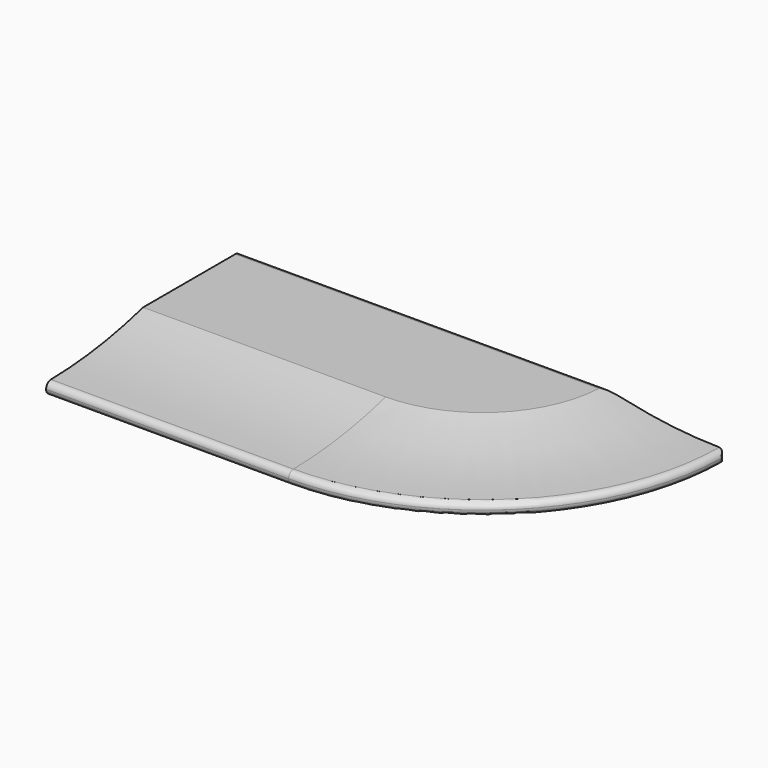
from build123d import *

# Parameters (mm, degrees)
F1_DEPTH     = 4.7625
F2_W         = 19.05
F2_H         = 6.35
F3_DEPTH     = 25.4
F4_R         = 2.54
F9_T1_DEPTH  = 9.0533559085
F9_T3_DEPTH  = 84.7725
F9_T5_DEPTH  = 53.9538612207
F9_T8_ANGLE  = 93.5585733653
F9_T10_ANGLE = 93.5585733653


# Not quite as in the source:
# - a fillet or chamfer that OpenCascade refuses, or shapes differently, is made with other operations: its cross-section is extruded or revolved along the edge and cut away or added
# - two fillets or chamfers of one size are made in one step


with BuildPart() as f1:
    # F0 (on Top) → F1 (new body, symmetric)
    with BuildSketch(Plane.XY):
        with BuildLine():
            Line((101.6, 0), (0, 0))
            Line((0, 0), (0, -50.8))
            Line((0, -50.8), (50.8, -50.8))
            ThreePointArc((50.8, -50.8), (86.7210244843, -35.9210244843), (101.6, 0))
        make_face()
    extrude(amount=F1_DEPTH, both=True)

    # F2 (on Right) → F3 (cut)
    with BuildSketch(Plane.YZ):
        with Locations((-12.7, 0)):
            Rectangle(F2_W, F2_H)
    extrude(amount=F3_DEPTH, mode=Mode.SUBTRACT)

    # F4
    f4_edges = [f1.edges().sort_by_distance(p)[0] for p in [
        (12.7, -3.175, -3.175),
        (12.7, -3.175, 3.175),
        (12.7, -22.225, -3.175),
        (12.7, -22.225, 3.175),
    ]]
    fillet(f4_edges, radius=F4_R)


with BuildPart() as f6:
    # F6: sweep along a path in F6_path
    with BuildLine(Plane(origin=(50.8, -50.8, 4.7625), x_dir=(0, 1, 0), z_dir=(0, 0, 1))) as f6_path:
        Line((0, 50.8), (0, 0))
        ThreePointArc((0, 0), (14.8789755157, -35.9210244843), (50.8, -50.8))
    # F5 (on face) → F6 (sweep)
    with BuildSketch(Plane(origin=(0, 0, 0), x_dir=(0, -1, 0), z_dir=(-1, 0, 0))):
        with BuildLine():
            Line((50.8, 4.7625), (25.4, 4.7625))
            ThreePointArc((25.4, 4.7625), (37.9805074569, 2.1472133229), (50.8, 1.27))
            Line((50.8, 1.27), (50.8, 4.7625))
        make_face()
    sweep(path=f6_path.line)


with BuildPart() as f7_1:
    # F7: instance of F6
    add(f6.part.mirror(Plane.XY))


with BuildPart() as f1_1:
    add(f1.part)

    # F8: cut F6, F7_1
    add(f6.part, mode=Mode.SUBTRACT)
    add(f7_1.part, mode=Mode.SUBTRACT)

    # F9: fillet of radius 1.27 on 8 edges, made by hand

    # F9_s2 → F9_t1 (cut)
    with BuildSketch(Plane.XY.offset(-4.5266779542)):
        with BuildLine():
            ThreePointArc((100.3137152716, 0), (101.2231811617, -0.3835623006), (101.5832977145, -1.3025641026))
            ThreePointArc((101.5832977145, -1.3025641026), (101.595824257, -0.6513355908), (101.6, 0))
            Line((101.6, 0), (100.3137152716, 0))
        make_face()
    extrude(amount=F9_T1_DEPTH, mode=Mode.SUBTRACT)

    # F9_s4 → F9_t3 (cut)
    with BuildSketch(Plane.YZ.offset(-3.175)):
        with BuildLine():
            ThreePointArc((0, 3.4925), (-0.3719743879, 4.3905256121), (-1.27, 4.7625))
            Line((-1.27, 4.7625), (0, 4.7625))
            Line((0, 4.7625), (0, 3.4925))
        make_face()
        with BuildLine():
            ThreePointArc((0, -3.4925), (-0.3719743879, -4.3905256121), (-1.27, -4.7625))
            Line((-1.27, -4.7625), (0, -4.7625))
            Line((0, -4.7625), (0, -3.4925))
        make_face()
    extrude(amount=F9_T3_DEPTH, mode=Mode.SUBTRACT)

    # F9_s6 → F9_t5 (cut)
    with BuildSketch(Plane.YZ.offset(-3.1538612207)):
        with BuildLine():
            ThreePointArc((-49.5469102739, 1.2783429251), (-50.4339845264, 0.9004824038), (-50.8, 0.0084555117))
            Line((-50.8, 0.0084555117), (-50.8, 1.27))
            ThreePointArc((-50.8, 1.27), (-50.1734412505, 1.2720857544), (-49.5469102739, 1.2783429251))
        make_face()
        with BuildLine():
            ThreePointArc((-50.8, -0.0084555117), (-50.4339845264, -0.9004824038), (-49.5469102739, -1.2783429251))
            ThreePointArc((-49.5469102739, -1.2783429251), (-50.1734412505, -1.2720857544), (-50.8, -1.27))
            Line((-50.8, -1.27), (-50.8, -0.0084555117))
        make_face()
    extrude(amount=F9_T5_DEPTH, mode=Mode.SUBTRACT)

    # F9_s7 → F9_t8 (revolve, cut)
    with BuildSketch(Plane.YZ.offset(50.8)):
        with BuildLine():
            ThreePointArc((-50.8, 0.0084555117), (-50.4339845264, 0.9004824038), (-49.5469102739, 1.2783429251))
            ThreePointArc((-49.5469102739, 1.2783429251), (-50.1734412505, 1.2720857544), (-50.8, 1.27))
            Line((-50.8, 1.27), (-50.8, 0.0084555117))
        make_face()
    revolve(axis=Axis((50.8, 0, 1.27), (0, 0, 1)), revolution_arc=F9_T8_ANGLE, mode=Mode.SUBTRACT)

    # F9_s9 → F9_t10 (revolve, cut)
    with BuildSketch(Plane.YZ.offset(50.8)):
        with BuildLine():
            ThreePointArc((-50.8, -0.0084555117), (-50.4339845264, -0.9004824038), (-49.5469102739, -1.2783429251))
            ThreePointArc((-49.5469102739, -1.2783429251), (-50.1734412505, -1.2720857544), (-50.8, -1.27))
            Line((-50.8, -1.27), (-50.8, -0.0084555117))
        make_face()
    revolve(axis=Axis((50.8, 0, -1.27), (0, 0, 1)), revolution_arc=F9_T10_ANGLE, mode=Mode.SUBTRACT)


solid = f1_1.part
